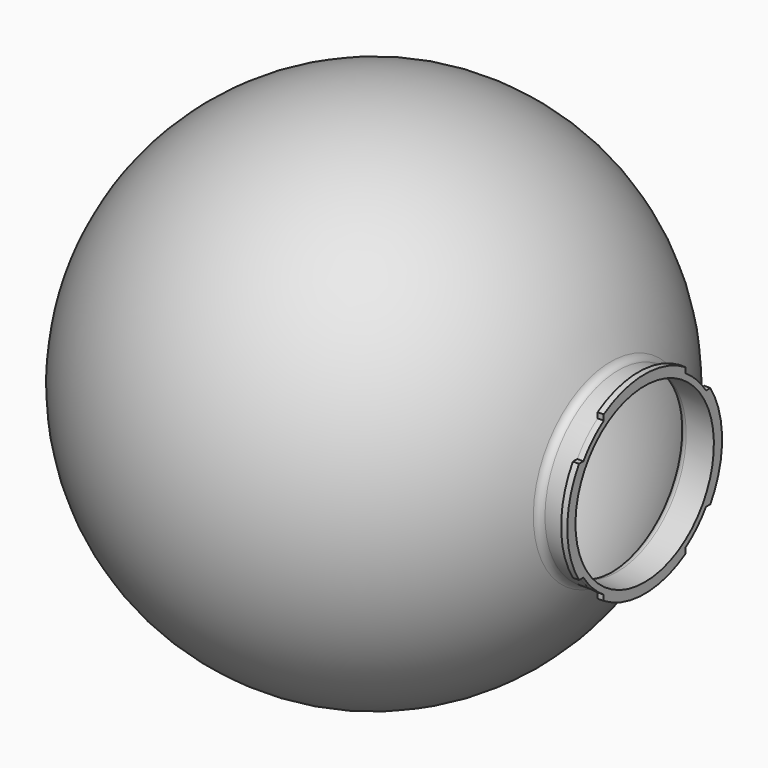
from build123d import *

# Parameters (mm, degrees)
F3_DEPTH = 25


with BuildPart() as f1:
    # F0 (on Front) → F1 (revolve)
    with BuildSketch(Plane.XZ):
        with BuildLine():
            ThreePointArc((230.1764353028, -89.5980392157), (-45.581906938, -242.757677036), (-247, 0))
            Line((-247, 0), (-250, 0))
            ThreePointArc((-250, 0), (-48.1392607307, -245.3214454064), (231.4608926104, -94.476744186))
            ThreePointArc((231.4608926104, -94.476744186), (234.4059176567, -90.8597422297), (238.8676411739, -89.5))
            Line((238.8676411739, -89.5), (258.6609246731, -89.5))
            Line((258.6609246731, -89.5), (258.6609246731, -94.5))
            Line((258.6609246731, -94.5), (264.6609246731, -94.5))
            Line((264.6609246731, -94.5), (264.6609246731, -84.5))
            Line((264.6609246731, -84.5), (237.6315425191, -84.5))
            ThreePointArc((237.6315425191, -84.5), (233.1157749362, -85.8963765146), (230.1764353028, -89.5980392157))
        make_face()
    revolve(axis=Axis((132.3304623365, 0, 0), (1, 0, 0)))

    # F2 (on face) → F3 (cut)
    with BuildSketch(Plane.YZ.offset(264.6609246731)):
        with BuildLine():
            ThreePointArc((50, 74.8331477355), (63.6396103068, 63.6396103068), (74.8331477355, 50))
            Line((74.8331477355, 50), (80.1888396225, 50))
            ThreePointArc((80.1888396225, 50), (66.8215908221, 66.8215908221), (50, 80.1888396225))
            Line((50, 80.1888396225), (50, 74.8331477355))
        make_face()
        with BuildLine():
            Line((80.1888396225, -50), (74.8331477355, -50))
            ThreePointArc((74.8331477355, -50), (63.6396103068, -63.6396103068), (50, -74.8331477355))
            Line((50, -74.8331477355), (50, -80.1888396225))
            ThreePointArc((50, -80.1888396225), (66.8215908221, -66.8215908221), (80.1888396225, -50))
        make_face()
        with BuildLine():
            Line((119.5877417922, 50), (80.1888396225, 50))
            ThreePointArc((80.1888396225, 50), (90.8517895925, 26.0038906289), (94.5, 0))
            ThreePointArc((94.5, 0), (90.8517895925, -26.0038906289), (80.1888396225, -50))
            Line((80.1888396225, -50), (119.5877417922, -50))
            Line((119.5877417922, -50), (119.5877417922, 50))
        make_face()
        with BuildLine():
            ThreePointArc((-74.8331477355, 50), (-63.6396103068, 63.6396103068), (-50, 74.8331477355))
            Line((-50, 74.8331477355), (-50, 80.1888396225))
            ThreePointArc((-50, 80.1888396225), (-66.8215908221, 66.8215908221), (-80.1888396225, 50))
            Line((-80.1888396225, 50), (-74.8331477355, 50))
        make_face()
        with BuildLine():
            Line((-50, -80.1888396225), (-50, -74.8331477355))
            ThreePointArc((-50, -74.8331477355), (-63.6396103068, -63.6396103068), (-74.8331477355, -50))
            Line((-74.8331477355, -50), (-80.1888396225, -50))
            ThreePointArc((-80.1888396225, -50), (-66.8215908221, -66.8215908221), (-50, -80.1888396225))
        make_face()
        with BuildLine():
            ThreePointArc((-80.1888396225, -50), (-94.5, 0), (-80.1888396225, 50))
            Line((-80.1888396225, 50), (-119.5877417922, 50))
            Line((-119.5877417922, 50), (-119.5877417922, -50))
            Line((-119.5877417922, -50), (-80.1888396225, -50))
        make_face()
    extrude(amount=-F3_DEPTH, mode=Mode.SUBTRACT)


solid = f1.part
